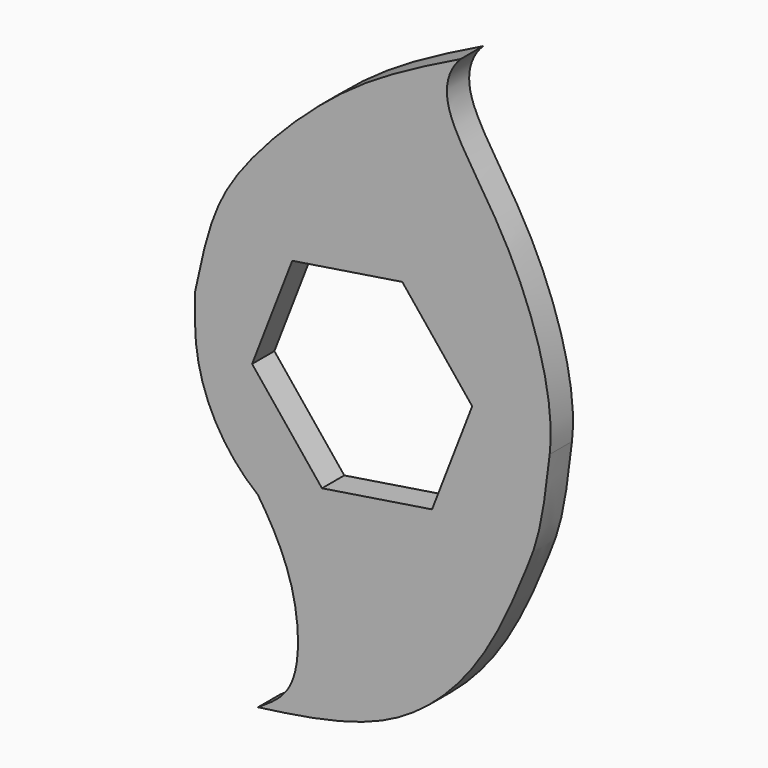
from build123d import *

# Parameters (mm, degrees)
F1_DEPTH = 5


with BuildPart() as f1:
    # F0 (on Front) → F1 (new body)
    with BuildSketch(Plane.XZ):
        with BuildLine():
            add(Edge.make_bspline(
                [(17.7268970846, 57.3215240529), (15.7368547016, 55.3111901481), (13.2864885412, 48.3492794063), (27.4724268838, 31.8894637146), (34.7996985334, 9.2238161581), (33.6772166193, 0)],
                knots=[0, 0, 0, 0, 0.0998215374, 0.2608171732, 0.4613817906, 0.4613817906, 0.4613817906, 0.4613817906], degree=3))
            add(Edge.make_bspline(
                [(-30, 5), (-29.0251400049, 9.6311227922), (-27.111556473, 18.7217002639), (-20.3931031734, 29.7414743972), (-3.0886979237, 47.0172460729), (10.8010188696, 53.8930285257), (17.7268970846, 57.3215240529)],
                knots=[0, 0, 0, 0, 0.217604872, 0.4271434889, 0.714354548, 1, 1, 1, 1], degree=3))
            Line((-30, 5), (-30, 0))
            ThreePointArc((-30, 0), (-27.0280044879, -13.0187162732), (-18.7008684399, -23.4579947906))
            add(Edge.make_bspline(
                [(-18.7008684399, -57.0112052109), (-16.3589078306, -55.4979023543), (-11.3874918945, -52.4259033179), (-11.0828909126, -37.6937310973), (-15.0989089292, -28.8739952525), (-18.7008684399, -23.4579947906)],
                knots=[0, 0, 0, 0, 0.2676818681, 0.6095268804, 1, 1, 1, 1], degree=3))
            add(Edge.make_bspline(
                [(33.6772166193, 0), (32.7849820148, -7.3317956016), (23.9235568427, -18.4163736638), (6.4508308138, -37.9844205648), (-6.683168554, -53.2337896345), (-18.7008684399, -57.0112052109)],
                knots=[0.4613817906, 0.4613817906, 0.4613817906, 0.4613817906, 0.6208059112, 0.8001995813, 1, 1, 1, 1], degree=3))
        make_face()
        Polygon((-12.5522075988, 15.5705518334), (7.2083896393, 18.6558065708), (19.7605972381, 3.0852547374), (12.5522075988, -15.5705518334), (-7.2083896393, -18.6558065708), (-19.7605972381, -3.0852547374), align=None, mode=Mode.SUBTRACT)
        with BuildLine():
            add(Edge.make_bspline(
                [(33.6772166193, 0), (32.2933898964, -12.6003254892), (30.2817412105, -17.4795691907), (22.1883431115, -37.3342070936), (6.1289464447, -53.5681106433), (-10.7206157713, -55.9326505298), (-18.7008684399, -57.0112052109)],
                knots=[0, 0, 0, 0, 0.243897848, 0.4755092955, 0.7316307838, 1, 1, 1, 1], degree=3))
            add(Edge.make_bspline(
                [(33.6772166193, 0), (32.7849820148, -7.3317956016), (23.9235568427, -18.4163736638), (6.4508308138, -37.9844205648), (-6.683168554, -53.2337896345), (-18.7008684399, -57.0112052109)],
                knots=[0.4613817906, 0.4613817906, 0.4613817906, 0.4613817906, 0.6208059112, 0.8001995813, 1, 1, 1, 1], degree=3))
        make_face()
    extrude(amount=F1_DEPTH)


solid = f1.part
